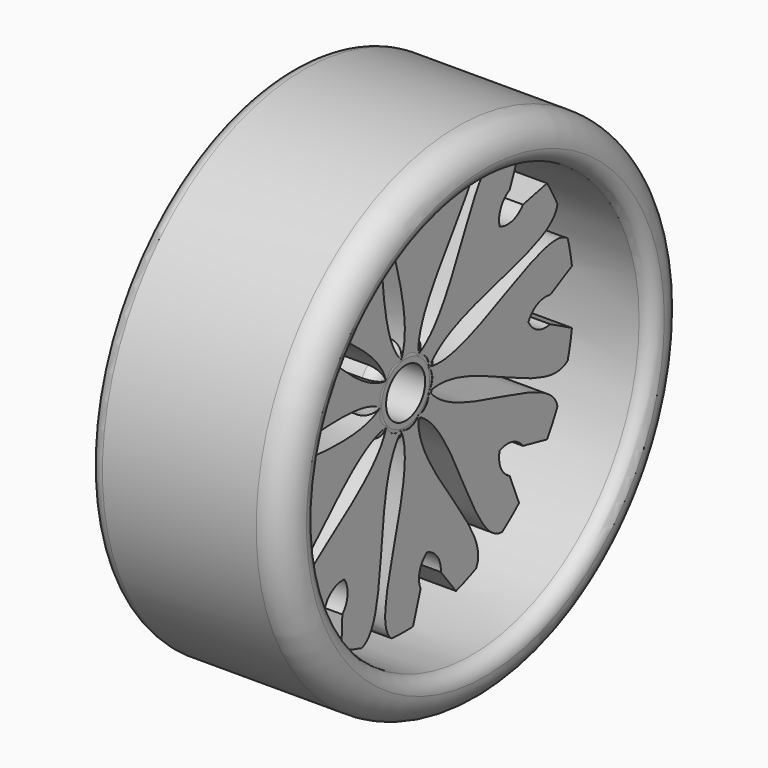
from build123d import *

# Parameters (mm, degrees)
F3_DEPTH = 5
F4_COUNT = 9


# Not quite as in the source:
# - ends of sketch curves that miss each other by under 0.0002 mm in the source are joined


with BuildPart() as f1:
    # F0 (on Top) → F1 (revolve)
    with BuildSketch(Plane.XY):
        with BuildLine():
            Line((0, 17), (0, 16.0000003735))
            ThreePointArc((0, 16.0000003735), (0.2928932188, 15.2928935923), (1, 15.0000003735))
            Line((1, 15.0000003735), (13, 15.0000003735))
            ThreePointArc((13, 15.0000003735), (13.7071067812, 15.2928935923), (14, 16.0000003735))
            ThreePointArc((14, 16.0000003735), (13.4142135624, 17.4142135624), (12, 18))
            Line((12, 18), (1, 18))
            ThreePointArc((1, 18), (0.2928932188, 17.7071067812), (0, 17))
        make_face()
    revolve(axis=Axis((-21.5144966841, 0, 0), (1, 0, 0)))



with BuildPart() as f1b:
    # F0 (on Top) → F1, piece 2 (revolve)
    with BuildSketch(Plane.XY):
        with BuildLine():
            Line((7.2954415227, 3.1500400949), (2, 3.1500400949))
            Line((2, 3.1500400949), (-2.2713001128, 3.1500400949))
            ThreePointArc((-2.2713001128, 3.1500400949), (-2.978406894, 2.8571468761), (-3.2713001128, 2.1500400949))
            Line((-3.2713001128, 2.1500400949), (-3.2713001128, 1.75))
            Line((-3.2713001128, 1.75), (8.2954415227, 1.75))
            Line((8.2954415227, 1.75), (8.2954415227, 2.1500400949))
            ThreePointArc((8.2954415227, 2.1500400949), (8.0025483039, 2.8571468761), (7.2954415227, 3.1500400949))
        make_face()
    revolve(axis=Axis((-21.5144966841, 0, 0), (1, 0, 0)))


with BuildPart() as f1_1:
    add(f1.part)

    add(f1b.part)  # F3 merges F1b
    # F2 (on face) → F3 (join)
    with BuildSketch(Plane.YZ.offset(8.2954415227)):
        with BuildLine():
            add(Edge.make_bspline(
                [(1.985329801, -0.825310845), (6.186098326, 0.5037762458), (14.9991028011, -7.9743831884), (15.0886839256, -2.0620899741)],
                knots=[0, 0, 0, 0, 13.1615923021, 13.1615923021, 13.1615923021, 13.1615923021], degree=3))
            Line((15.0886839256, -2.0620899741), (12.9203172401, -0.920843333))
            ThreePointArc((12.9203172401, -0.920843333), (11.7871554884, -0.804062332), (10.9802000225, 0))
            ThreePointArc((10.9802000225, 0), (11.7871554884, 0.804062332), (12.9203172401, 0.920843333))
            Line((12.9203172401, 0.920843333), (15.0886839256, 2.0620899741))
            add(Edge.make_bspline(
                [(1.985329801, 0.825310845), (6.186098326, -0.5037762458), (14.9991028011, 7.9743831884), (15.0886839256, 2.0620899741)],
                knots=[0, 0, 0, 0, 13.1615923021, 13.1615923021, 13.1615923021, 13.1615923021], degree=3))
            ThreePointArc((1.985329801, 0.825310845), (2.3855323046, 0), (1.985329801, -0.825310845))
        make_face()
    extrude(amount=-F3_DEPTH)

    # F4: F1 ×9 about axis
    f4_axis = Axis((14, 0, 0), (1, 0, 0))


with BuildPart() as f1_2:
    add(f1_1.part)
    for i in range(1, F4_COUNT):
        add(f1_1.part.rotate(f4_axis, i * 360 / F4_COUNT))


solid = f1_2.part
